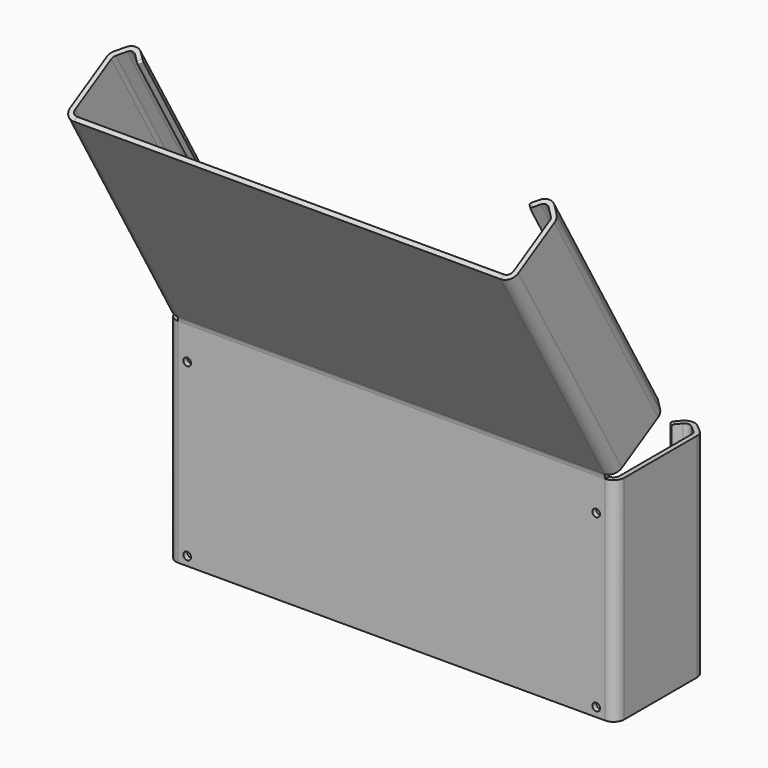
from build123d import *

# Parameters (mm, degrees)
F1_DEPTH  = 74.8970308
F2_R      = 1.35255
F3_DEPTH  = 1.70942
F8_DEPTH  = 150.2936248359
F10_DEPTH = 91.0812758
F11_R     = 3.69315
F12_R     = 1.98373
F12_R_2   = 1.98374
F13_R     = 0.762


# Not quite as in the source:
# - a fillet or chamfer is up to 0.001 mm smaller than in the source, because OpenCascade refuses the exact size


with BuildPart() as f1:
    # F0 (on Top) → F1 (new body)
    with BuildSketch(Plane.XY):
        Polygon((0, -34.9127429517), (0, 0), (4.6326774961, 3.932751029), (7.9712502047, 0), (9.2744217668, 1.1062823402), (4.8295667179, 6.3422049313), (-1.70942, 0.7911587457), (-1.70942, -36.6221629517), (155.9705248359, -36.6221629517), (155.9705248359, 0.7911587457), (149.4315381179, 6.3422049313), (144.9866830691, 1.1062823402), (146.2898546311, 0), (149.6284273398, 3.932751029), (154.2611048359, 0), (154.2611048359, -34.9127429517), align=None)
    extrude(amount=F1_DEPTH)

    # F2 (on face) → F3 (cut, through all)
    with BuildSketch(Plane(origin=(0, -34.9127429517, 0), x_dir=(-1, 0, 0), z_dir=(0, 1, 0))):
        with Locations((-5.15874, 3.175)):
            Circle(F2_R)
        with Locations((-5.15874, 63.2981208)):
            Circle(F2_R)
        with Locations((-149.1023648359, 63.2981208)):
            Circle(F2_R)
        with Locations((-149.1023648359, 3.175)):
            Circle(F2_R)
    extrude(amount=-F3_DEPTH, mode=Mode.SUBTRACT)

    # F7 (on offset) → F8 (join, through all)
    with BuildSketch(Plane.YZ.offset(1.98374)):
        with BuildLine():
            Line((-36.6221629517, 74.8970308), (-34.9127429517, 74.8970308))
            ThreePointArc((-34.9127429517, 74.8970308), (-35.0846656967, 76.2029136969), (-35.5887176805, 77.4198028324))
            Line((-35.5887176805, 77.4198028324), (-81.129350806, 156.2984932146))
            Line((-81.129350806, 156.2984932146), (-82.6097519517, 155.4437832146))
            Line((-82.6097519517, 155.4437832146), (-37.0691188262, 76.5650928324))
            ThreePointArc((-37.0691188262, 76.5650928324), (-36.7358386226, 75.7604832448), (-36.6221629517, 74.8970308))
        make_face()
    extrude(amount=F8_DEPTH)

    # F9 (on face) → F10 (join)
    with BuildSketch(Plane(origin=(0, -87.96157055, 152.3539093062), x_dir=(1, 0, 0), z_dir=(0, -0.5, 0.8660254038))):
        Polygon((-1.7094199999, 6.1797478168), (1.98374, 6.1797478168), (1.98374, 7.8891678168), (0, 7.8891678168), (1e-10, 28.9964815425), (4.3557372213, 33.3522187635), (8.0035172575, 29.7044387269), (9.2122597315, 30.9131812007), (4.3557372215, 35.7697037112), (-1.7094199999, 29.7045464903), align=None)
        Polygon((152.277364836, 7.8891678168), (152.277364836, 6.1797478168), (155.9705248359, 6.1797478168), (155.9705248359, 29.7045464903), (149.9053676148, 35.7697037114), (145.0488451045, 30.9131812012), (146.2575875784, 29.7044387273), (149.9053676148, 33.3522187636), (154.2611048359, 28.9964815425), (154.2611048359, 7.8891678168), align=None)
    extrude(amount=-F10_DEPTH)

    # F11 (radius 3.69316 in the source; OpenCascade refuses exactly that, so slightly less here)
    f11_edges = [f1.edges().sort_by_distance(p)[0] for p in [
        (149.431538, 6.342205, 37.448515),
        (155.970525, 0.791159, 37.448515),
        (155.970525, -36.622163, 37.448515),
        (-1.70942, -36.622163, 37.448515),
        (-1.70942, 0.791159, 37.448515),
        (4.829567, 6.342205, 37.448515),
        (149.905368, -34.21378, 130.799412),
        (155.970525, -39.46636, 127.766833),
        (155.970525, -59.839433, 116.004434),
        (-1.70942, -59.839433, 116.004434),
        (-1.70942, -39.46636, 127.766833),
        (4.355737, -34.21378, 130.799412),
    ]]
    fillet(f11_edges, radius=F11_R)

    # F12#9 (call 1 of 12: OpenCascade refuses the feature's edges together) (radius 1.98374 in the source; OpenCascade refuses exactly that, so slightly less here)
    f12_9_edges = [f1.edges().sort_by_distance(p)[0] for p in [
        (0, -58.359032, 116.859144),
    ]]
    fillet(f12_9_edges, radius=F12_R)

    # F12#10 (call 2 of 12) (radius 1.98374 in the source; OpenCascade refuses exactly that, so slightly less here)
    f12_10_edges = [f1.edges().sort_by_distance(p)[0] for p in [
        (154.261105, -58.359032, 116.859144),
    ]]
    fillet(f12_10_edges, radius=F12_R)

    # F12#11 (call 3 of 12)
    f12_11_edges = [f1.edges().sort_by_distance(p)[0] for p in [
        (154.261105, -40.079562, 127.412801),
    ]]
    fillet(f12_11_edges, radius=F12_R_2)

    # F12#12 (call 4 of 12)
    f12_12_edges = [f1.edges().sort_by_distance(p)[0] for p in [
        (149.905368, -36.307383, 129.590669),
    ]]
    fillet(f12_12_edges, radius=F12_R_2)

    # F12 (call 5 of 12)
    f12_edges = [f1.edges().sort_by_distance(p)[0] for p in [
        (149.628427, 3.932751, 37.448515),
    ]]
    fillet(f12_edges, radius=F12_R_2)

    # F12#2 (call 6 of 12)
    f12_2_edges = [f1.edges().sort_by_distance(p)[0] for p in [
        (154.261105, 0, 37.448515),
    ]]
    fillet(f12_2_edges, radius=F12_R_2)

    # F12#3 (call 7 of 12)
    f12_3_edges = [f1.edges().sort_by_distance(p)[0] for p in [
        (154.261105, -34.912743, 37.448515),
    ]]
    fillet(f12_3_edges, radius=F12_R_2)

    # F12#4 (call 8 of 12)
    f12_4_edges = [f1.edges().sort_by_distance(p)[0] for p in [
        (0, -34.912743, 37.448515),
    ]]
    fillet(f12_4_edges, radius=F12_R_2)

    # F12#5 (call 9 of 12)
    f12_5_edges = [f1.edges().sort_by_distance(p)[0] for p in [
        (0, 0, 37.448515),
    ]]
    fillet(f12_5_edges, radius=F12_R_2)

    # F12#6 (call 10 of 12)
    f12_6_edges = [f1.edges().sort_by_distance(p)[0] for p in [
        (4.632677, 3.932751, 37.448515),
    ]]
    fillet(f12_6_edges, radius=F12_R_2)

    # F12#7 (call 11 of 12)
    f12_7_edges = [f1.edges().sort_by_distance(p)[0] for p in [
        (0, -40.079562, 127.412801),
    ]]
    fillet(f12_7_edges, radius=F12_R_2)

    # F12#8 (call 12 of 12)
    f12_8_edges = [f1.edges().sort_by_distance(p)[0] for p in [
        (4.355737, -36.307383, 129.590669),
    ]]
    fillet(f12_8_edges, radius=F12_R_2)

    # F13
    f13_edges = [f1.edges().sort_by_distance(p)[0] for p in [
        (145.638269, 0.553141, 74.897031),
        (145.638269, 0.553141, 0),
        (8.622836, 0.553141, 0),
        (8.622836, 0.553141, 74.897031),
        (8.607888, -61.713371, 167.508314),
        (8.607888, -16.172733, 88.629616),
        (145.653216, -16.172733, 88.629616),
        (145.653216, -61.713371, 167.508314),
    ]]
    fillet(f13_edges, radius=F13_R)


solid = f1.part
